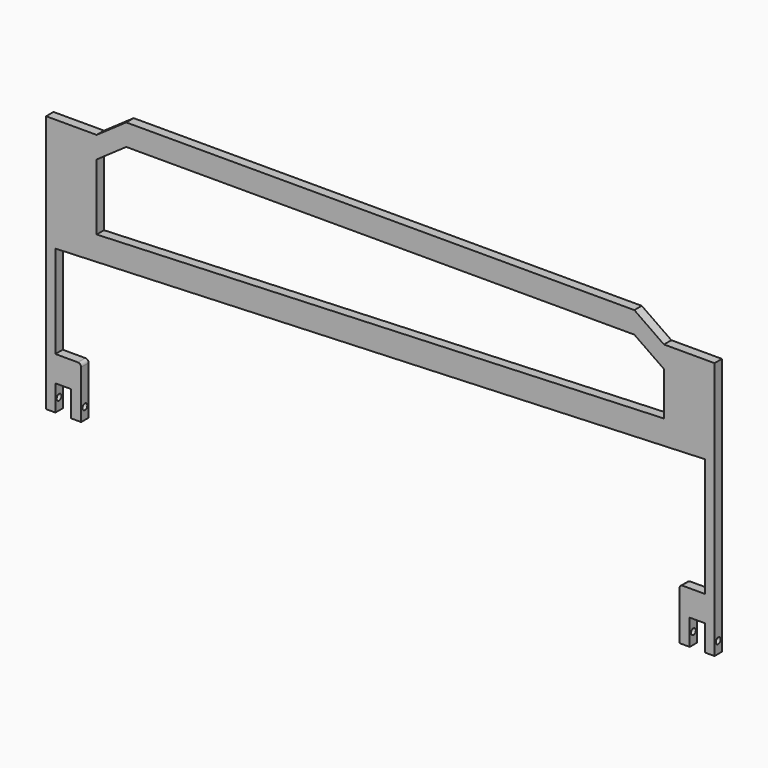
from build123d import *

# Parameters (mm, degrees)
F1_DEPTH = 9
F2_R     = 5.8193233161
F3_DEPTH = 1800


# Not quite as in the source:
# - a feature names something its author has since deleted; it is built from what else it names


with BuildPart() as f1:
    # F0 (on Front) → F1 (new body, symmetric)
    with BuildSketch(Plane.XZ):
        with BuildLine():
            Line((492.5543735346, 210), (0, 210))
            Line((0, 210), (-492.5543735346, 210))
            Line((-492.5543735346, 210), (-550, 170))
            Line((-550, 170), (-630, 170))
            Line((-630, 170), (-648, 170))
            Line((-648, 170), (-648, -230))
            Line((-648, -230), (-648, -330))
            Line((-648, -330), (-630, -330))
            Line((-630, -330), (-630, -280))
            Line((-630, -280), (-600, -280))
            Line((-600, -280), (-600, -330))
            Line((-600, -330), (-580, -330))
            Line((-580, -330), (-580, -236.35))
            ThreePointArc((-580, -236.35), (-581.8598719395, -231.8598719395), (-586.35, -230))
            Line((-586.35, -230), (-630, -230))
            Line((-630, -230), (-630, -50))
            Line((-630, -50), (630, 0))
            Line((630, 0), (630, -50))
            Line((630, -50), (630, -230))
            Line((630, -230), (586.35, -230))
            ThreePointArc((586.35, -230), (581.8598719395, -231.8598719395), (580, -236.35))
            Line((580, -236.35), (580, -330))
            Line((580, -330), (600, -330))
            Line((600, -330), (600, -280))
            Line((600, -280), (630, -280))
            Line((630, -280), (630, -330))
            Line((630, -330), (648, -330))
            Line((648, -330), (648, -230))
            Line((648, -230), (648, 170))
            Line((648, 170), (630, 170))
            Line((630, 170), (550, 170))
            Line((550, 170), (492.5543735346, 210))
        make_face()
        Polygon((550, 43.6507936508), (-550, 0), (-550, 128.1044334173), (-492.5543735346, 168.1044334173), (492.5543735346, 168.1044334173), (550, 128.1044334173), align=None, mode=Mode.SUBTRACT)
    extrude(amount=F1_DEPTH, both=True)

    # F2 (on face) → F3 (cut)
    with BuildSketch(Plane.YZ.offset(648)):
        with Locations((0, -307.489156723)):
            Circle(F2_R)
    extrude(amount=-F3_DEPTH, mode=Mode.SUBTRACT)


solid = f1.part
